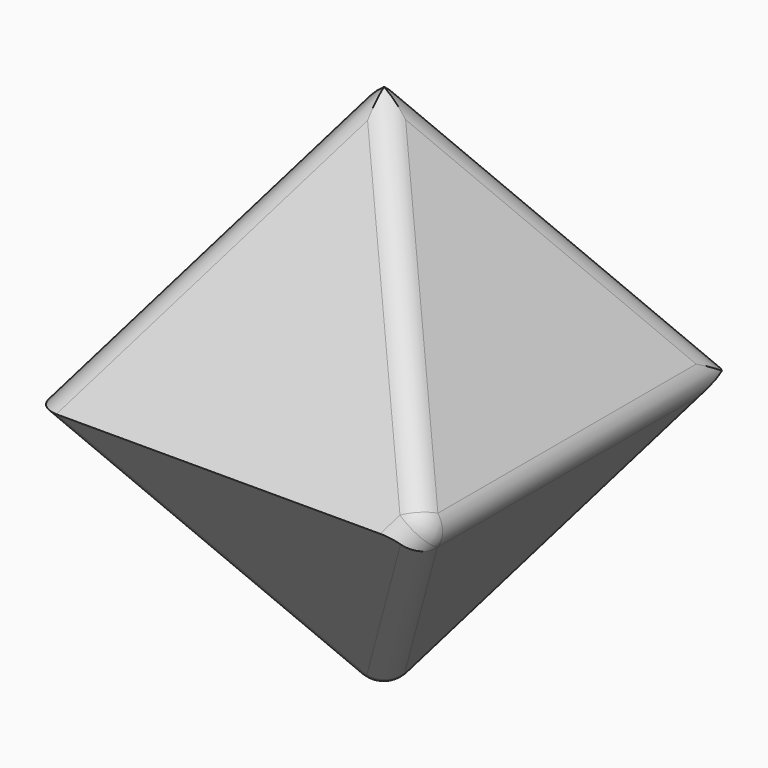
from build123d import *

# Parameters (mm, degrees)
F0_W          = 15
F0_H          = 15
F1_DEPTH      = 30
F1_DEPTH_BACK = 25
F3_DEPTH      = 61.89487
F5_DEPTH      = 47.86065
F6_T1_DEPTH   = 15.5059160489
F6_T3_DEPTH   = 15.4680372972
F6_T5_DEPTH   = 3.5726399386
F6_T7_DEPTH   = 15.5059160489
F6_T9_DEPTH   = 0.0371060326
F6_T11_DEPTH  = 15.5055296894
F6_T13_DEPTH  = 18.4976551542
F6_T15_DEPTH  = 18.4904222245
F6_T17_DEPTH  = 15.4680372972
F6_T19_DEPTH  = 15.5059160489
F6_T21_DEPTH  = 18.4904222245
F6_T26_DEPTH  = 2.1200301885
F6_S37_W      = 4.2400603769
F6_S37_H      = 4.2400603769
F6_T38_DEPTH  = 2.1200301885
F6_S49_W      = 4.2400603769
F6_S49_H      = 4.2400603769
F6_T50_DEPTH  = 2.1200301885


# Not quite as in the source:
# - a fillet or chamfer that OpenCascade refuses, or shapes differently, is made with other operations: its cross-section is extruded or revolved along the edge and cut away or added


with BuildPart() as f1:
    # F0 (on Top) → F1 (new body, two sides)
    with BuildSketch(Plane.XY) as f1_sk:
        with Locations((-36.2346637994, 35.6825158745)):
            Rectangle(F0_W, F0_H)
    extrude(amount=F1_DEPTH)
    extrude(f1_sk.sketch, amount=-F1_DEPTH_BACK)

    # F2 (on Right) → F3 (cut)
    with BuildSketch(Plane.YZ):
        Polygon((56.5448105335, -31.7836888134), (61.0591061413, 3.6857917439), (59.3393743038, 37.8654710948), (23.6549284309, 37.8654710948), (21.0753269494, -33.503420651), align=None)
        Polygon((35.7014552504, 20.6066017178), (43.2014552504, 10), (35.7014552504, -0.6066017178), (28.2014552504, 10), align=None, mode=Mode.SUBTRACT)
    extrude(amount=-F3_DEPTH, mode=Mode.SUBTRACT)

    # F4 (on Front) → F5 (cut)
    with BuildSketch(Plane.XZ):
        Polygon((-47.5901886821, 22.4271342158), (-47.5901886821, -2.1975641139), (-25.7775690407, -2.0455596969), (-25.7775690407, 22.4271342158), align=None)
        Polygon((-36.2386666238, 20.6328396451), (-28.7386666238, 10.0262379273), (-36.2386666238, -0.5803637905), (-43.7386666238, 10.0262379273), align=None, mode=Mode.SUBTRACT)
    extrude(amount=-F5_DEPTH, mode=Mode.SUBTRACT)

    # F6: fillet of radius 1 on 12 edges, made by hand

    # F6_s2 → F6_t1 (cut)
    with BuildSketch(Plane(origin=(-18.3968515724, 18.3968515724, 26.0170769987), x_dir=(-0.7071067812, -0.7071067812, 0), z_dir=(-0.5, 0.5, 0.7071067812))):
        with BuildLine():
            ThreePointArc((0.9440971106, -21.7979649076), (0.3667468414, -21.6144614885), (-0.2106034277, -21.7979649076))
            Line((-0.2106034277, -21.7979649076), (0.3667468414, -21.3897166171))
            Line((0.3667468414, -21.3897166171), (0.9440971106, -21.7979649076))
        make_face()
    extrude(amount=F6_T1_DEPTH, mode=Mode.SUBTRACT)

    # F6_s4 → F6_t3 (cut)
    with BuildSketch(Plane(origin=(8.0115369091, 8.0115369091, 11.3300241523), x_dir=(0.7071067812, -0.7071067812, 0), z_dir=(-0.5, -0.5, -0.7071067812))):
        with BuildLine():
            ThreePointArc((-50.3051167111, 0.2571982972), (-50.8824669803, 0.0736948781), (-51.4598172495, 0.2571982972))
            Line((-51.4598172495, 0.2571982972), (-50.8824669803, -0.1510499933))
            Line((-50.8824669803, -0.1510499933), (-50.3051167111, 0.2571982972))
        make_face()
    extrude(amount=F6_T3_DEPTH, mode=Mode.SUBTRACT)

    # F6_s6 → F6_t5 (cut)
    with BuildSketch(Plane(origin=(1.6288258555, 1.6288258555, 2.3035076156), x_dir=(-0.7071067812, 0.7071067812, 0), z_dir=(0.5, 0.5, 0.7071067812))):
        with BuildLine():
            ThreePointArc((41.4305658009, 8.1654465877), (41.0079160701, 7.3489500067), (41.4305658009, 6.5324534258))
            Line((41.4305658009, 6.5324534258), (40.2758652625, 7.3489500067))
            Line((40.2758652625, 7.3489500067), (41.4305658009, 8.1654465877))
        make_face()
    extrude(amount=F6_T5_DEPTH, mode=Mode.SUBTRACT)

    # F6_s8 → F6_t7 (cut)
    with BuildSketch(Plane(origin=(-17.5732093647, 17.5732093647, -24.852271018), x_dir=(0.7071067812, 0.7071067812, 0), z_dir=(0.5, -0.5, 0.7071067812))):
        with BuildLine():
            ThreePointArc((0.1843655004, 35.9586535476), (-0.3929847687, 35.7751501285), (-0.9703350379, 35.9586535476))
            Line((-0.9703350379, 35.9586535476), (-0.3929847687, 35.5504052571))
            Line((-0.3929847687, 35.5504052571), (0.1843655004, 35.9586535476))
        make_face()
    extrude(amount=F6_T7_DEPTH, mode=Mode.SUBTRACT)

    # F6_s10 → F6_t9 (cut)
    with BuildSketch(Plane.XZ.offset(-35.7200082667)):
        with BuildLine():
            ThreePointArc((-37.0551632048, 0.5743367479), (-36.2386666238, 0.1516870171), (-35.4221700429, 0.5743367479))
            Line((-35.4221700429, 0.5743367479), (-36.2386666238, -0.5803637905))
            Line((-36.2386666238, -0.5803637905), (-37.0551632048, 0.5743367479))
        make_face()
    extrude(amount=F6_T9_DEPTH, mode=Mode.SUBTRACT)

    # F6_s12 → F6_t11 (cut)
    with BuildSketch(Plane.XZ.offset(-44.9502828275)):
        with BuildLine():
            ThreePointArc((-29.1469149143, 10.6035881965), (-28.9634114952, 10.0262379273), (-29.1469149143, 9.4488876581))
            Line((-29.1469149143, 9.4488876581), (-28.7386666238, 10.0262379273))
            Line((-28.7386666238, 10.0262379273), (-29.1469149143, 10.6035881965))
        make_face()
    extrude(amount=F6_T11_DEPTH, mode=Mode.SUBTRACT)

    # F6_s14 → F6_t13 (cut)
    with BuildSketch(Plane(origin=(-8.2990819717, -8.2990819717, 11.7366742796), x_dir=(-0.7071067812, 0.7071067812, 0), z_dir=(0.5, 0.5, -0.7071067812))):
        with BuildLine():
            ThreePointArc((51.4335793222, 13.9034903428), (50.856229053, 14.0869937619), (50.2788787838, 13.9034903428))
            Line((50.2788787838, 13.9034903428), (50.856229053, 14.3117386333))
            Line((50.856229053, 14.3117386333), (51.4335793222, 13.9034903428))
        make_face()
    extrude(amount=F6_T13_DEPTH, mode=Mode.SUBTRACT)

    # F6_s16 → F6_t15 (cut)
    with BuildSketch(Plane(origin=(-19.0654624524, 19.0654624524, -26.9626355732), x_dir=(0.7071067812, 0.7071067812, 0), z_dir=(0.5, -0.5, 0.7071067812))):
        with BuildLine():
            ThreePointArc((-0.9703350379, 50.1421569667), (-0.3929847687, 50.3256603857), (0.1843655004, 50.1421569667))
            Line((0.1843655004, 50.1421569667), (-0.3929847687, 50.5504052571))
            Line((-0.3929847687, 50.5504052571), (-0.9703350379, 50.1421569667))
        make_face()
    extrude(amount=F6_T15_DEPTH, mode=Mode.SUBTRACT)

    # F6_s18 → F6_t17 (cut)
    with BuildSketch(Plane(origin=(-18.3968515724, 18.3968515724, 26.0170769987), x_dir=(-0.7071067812, -0.7071067812, 0), z_dir=(-0.5, 0.5, 0.7071067812))):
        with BuildLine():
            ThreePointArc((0.9440971106, -35.9814683266), (0.3667468414, -36.1649717457), (-0.2106034277, -35.9814683266))
            Line((-0.2106034277, -35.9814683266), (0.3667468414, -36.3897166171))
            Line((0.3667468414, -36.3897166171), (0.9440971106, -35.9814683266))
        make_face()
    extrude(amount=F6_T17_DEPTH, mode=Mode.SUBTRACT)

    # F6_s20 → F6_t19 (cut)
    with BuildSketch(Plane(origin=(-8.2990819717, -8.2990819717, 11.7366742796), x_dir=(-0.7071067812, 0.7071067812, 0), z_dir=(0.5, 0.5, -0.7071067812))):
        with BuildLine():
            ThreePointArc((51.4335793222, -0.2800130762), (50.856229053, -0.4635164953), (50.2788787838, -0.2800130762))
            Line((50.2788787838, -0.2800130762), (50.856229053, -0.6882613667))
            Line((50.856229053, -0.6882613667), (51.4335793222, -0.2800130762))
        make_face()
    extrude(amount=F6_T19_DEPTH, mode=Mode.SUBTRACT)

    # F6_s22 → F6_t21 (cut)
    with BuildSketch(Plane(origin=(8.030476285, 8.030476285, 11.3568084745), x_dir=(0.7071067812, -0.7071067812, 0), z_dir=(-0.5, -0.5, -0.7071067812))):
        with BuildLine():
            ThreePointArc((-50.3051167111, 14.4407017163), (-50.8824669803, 14.6242051354), (-51.4598172495, 14.4407017163))
            Line((-51.4598172495, 14.4407017163), (-50.8824669803, 14.8489500067))
            Line((-50.8824669803, 14.8489500067), (-50.3051167111, 14.4407017163))
        make_face()
    extrude(amount=F6_T21_DEPTH, mode=Mode.SUBTRACT)


with BuildPart() as f6_tool24:
    # F6_s25 → F6_t26 (new body)
    with BuildSketch(Plane(origin=(-29.9207110183, 14.9603555092, -10.5785688295), x_dir=(0.4472135955, 0.894427191, 0), z_dir=(0.8528028654, -0.4264014327, 0.3015113446))):
        Polygon((12.2154363429, 24.5207679128), (10.0258785793, 20.8897971335), (13.6568493586, 18.7002393699), (15.8464071222, 22.3312101492), align=None)
    extrude(amount=F6_T26_DEPTH)

    split(bisect_by=Plane(origin=(-18.3968515724, 18.3968515724, 26.0170769987), x_dir=(0.7071067812, 0.7071067812, 0), z_dir=(0.5, -0.5, -0.7071067812)), keep=Keep.TOP)

    split(bisect_by=Plane.XZ.offset(-29.4447531381), keep=Keep.TOP)

    split(bisect_by=Plane(origin=(3.4151458248, 3.4151458248, 4.8297455429), x_dir=(-0.7071067812, 0.7071067812, 0), z_dir=(0.5, 0.5, 0.7071067812)), keep=Keep.TOP)

    split(bisect_by=Plane(origin=(0, 14.0705950274, -9.9494131592), x_dir=(1, 0, 0), z_dir=(0, 0.8164965809, -0.5773502692)), keep=Keep.TOP)

    split(bisect_by=Plane(origin=(-14.4163672655, 0, -10.1939110535), x_dir=(0, 1, 0), z_dir=(-0.8164965809, 0, -0.5773502692)), keep=Keep.TOP)

    split(bisect_by=Plane(origin=(-23.8691950364, 0, 16.8780696717), x_dir=(0, 1, 0), z_dir=(-0.8164965809, 0, 0.5773502692)), keep=Keep.TOP)

    # F6_s33 → F6_t34 (revolve, cut)
    with BuildSketch(Plane(origin=(-29.9634114952, 29.4447531381, 10.0262379273), x_dir=(-0.8528028654, 0.4264014327, -0.3015113446), z_dir=(-0.5222329679, -0.6963106238, 0.4923659639))):
        with BuildLine():
            ThreePointArc((0, -1), (1, 0), (0, 1))
            Line((0, 1), (0, -1))
        make_face()
    revolve(axis=Axis((-29.9634114952, 29.4447531381, 10.0262379273), (0, -0.5773502692, -0.8164965809)), mode=Mode.SUBTRACT)


with BuildPart() as f1_1:
    add(f1.part)

    # F6_t23: cut F6_tool24
    add(f6_tool24.part, mode=Mode.SUBTRACT)


with BuildPart() as f6_tool36:
    # F6_s37 → F6_t38 (new body)
    with BuildSketch(Plane(origin=(0, 6.0503474851, -12.8347252057), x_dir=(1, 0, 0), z_dir=(0, 0.4264014327, -0.9045340337))):
        with Locations((-36.2386666239, -32.8010441565)):
            Rectangle(F6_S37_W, F6_S37_H)
    extrude(amount=F6_T38_DEPTH)

    split(bisect_by=Plane(origin=(-18.3968515724, 18.3968515724, 26.0170769987), x_dir=(0.7071067812, 0.7071067812, 0), z_dir=(0.5, -0.5, -0.7071067812)), keep=Keep.TOP)

    split(bisect_by=Plane.XZ.offset(-35.7200082667), keep=Keep.BOTTOM)

    split(bisect_by=Plane(origin=(0.2775182605, 0.2775182605, 0.3924700878), x_dir=(0.7071067812, -0.7071067812, 0), z_dir=(-0.5, -0.5, -0.7071067812)), keep=Keep.TOP)

    split(bisect_by=Plane(origin=(0, 24.1032548906, -17.0435749818), x_dir=(1, 0, 0), z_dir=(0, -0.8164965809, 0.5773502692)), keep=Keep.TOP)

    split(bisect_by=Plane(origin=(-24.4490271287, 0, -17.2880728761), x_dir=(0, 1, 0), z_dir=(0.8164965809, 0, 0.5773502692)), keep=Keep.TOP)

    split(bisect_by=Plane(origin=(-23.8691950364, 0, 16.8780696717), x_dir=(0, 1, 0), z_dir=(-0.8164965809, 0, 0.5773502692)), keep=Keep.TOP)

    # F6_s45 → F6_t46 (revolve, cut)
    with BuildSketch(Plane(origin=(-36.2386666238, 35.7200082667, 1.1516870171), x_dir=(0, -0.4264014327, 0.9045340337), z_dir=(0, 0.9045340337, 0.4264014327))):
        with BuildLine():
            ThreePointArc((0, -1), (1, 0), (0, 1))
            Line((0, 1), (0, -1))
        make_face()
    revolve(axis=Axis((-36.2386666238, 35.7200082667, 1.1516870171), (1, 0, 0)), mode=Mode.SUBTRACT)


with BuildPart() as f1_2:
    add(f1_1.part)

    # F6_t35: cut F6_tool36
    add(f6_tool36.part, mode=Mode.SUBTRACT)


with BuildPart() as f6_tool48:
    # F6_s49 → F6_t50 (new body)
    with BuildSketch(Plane(origin=(0, 6.9319998787, 14.7049923642), x_dir=(1, 0, 0), z_dir=(0, -0.4264014327, -0.9045340337))):
        with Locations((-36.2386666239, -31.7853184989)):
            Rectangle(F6_S49_W, F6_S49_H)
    extrude(amount=F6_T50_DEPTH)

    split(bisect_by=Plane(origin=(-0.5461239472, -0.5461239472, 0.7723358929), x_dir=(-0.7071067812, 0.7071067812, 0), z_dir=(0.5, 0.5, -0.7071067812)), keep=Keep.TOP)

    split(bisect_by=Plane.XZ.offset(-35.6829022341), keep=Keep.TOP)

    split(bisect_by=Plane(origin=(-17.5732093647, 17.5732093647, -24.852271018), x_dir=(-0.7071067812, -0.7071067812, 0), z_dir=(-0.5, 0.5, -0.7071067812)), keep=Keep.TOP)

    split(bisect_by=Plane(origin=(0, 23.4986854432, 16.6160798259), x_dir=(1, 0, 0), z_dir=(0, 0.8164965809, 0.5773502692)), keep=Keep.TOP)

    split(bisect_by=Plane(origin=(-24.4490271287, 0, -17.2880728761), x_dir=(0, 1, 0), z_dir=(0.8164965809, 0, 0.5773502692)), keep=Keep.TOP)

    split(bisect_by=Plane(origin=(-23.8691950364, 0, 16.8780696717), x_dir=(0, 1, 0), z_dir=(-0.8164965809, 0, 0.5773502692)), keep=Keep.TOP)

    # F6_s57 → F6_t58 (revolve, cut)
    with BuildSketch(Plane(origin=(-36.2386666238, 35.6829022341, 1.1516870171), x_dir=(0, 0.4264014327, 0.9045340337), z_dir=(0, -0.9045340337, 0.4264014327))):
        with BuildLine():
            ThreePointArc((0, -1), (1, 0), (0, 1))
            Line((0, 1), (0, -1))
        make_face()
    revolve(axis=Axis((-36.2386666238, 35.6829022341, 1.1516870171), (-1, 0, 0)), mode=Mode.SUBTRACT)


with BuildPart() as f1_3:
    add(f1_2.part)

    # F6_t47: cut F6_tool48
    add(f6_tool48.part, mode=Mode.SUBTRACT)


solid = f1_3.part
